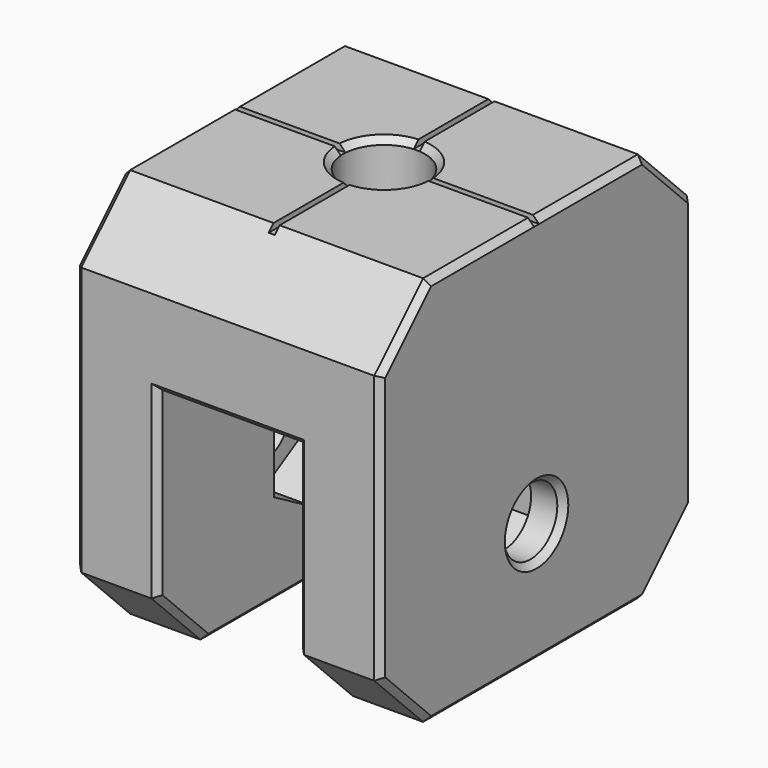
from build123d import *

# Parameters (mm, degrees)
F0_W      = 6.75
F0_H      = 32
F0_W_2    = 11.5
F0_R      = 3.35
F1_DEPTH  = 12
F2_DEPTH  = 20
F3_SIZE   = 5
F4_SIZE   = 5
F6_D      = 5.5
F8_DEPTH  = 4.1
F10_SIZE  = 0.5
F9_W      = 12.25
F9_H      = 0.5
F9_W_2    = 0.5
F9_H_2    = 15.75
F11_DEPTH = 0.5


# Not quite as in the source:
# - a pattern or mirror of a feature is missing from the dataset's text; its kind, count and spacing are read off the source's solid


with BuildPart() as f1:
    # F0 (on Top) → F1 (new body)
    with BuildSketch(Plane.XY):
        with Locations((9.125, 0)):
            Rectangle(F0_W, F0_H)
        Rectangle(F0_W_2, F0_H)
        Circle(F0_R, mode=Mode.SUBTRACT)
        with Locations((-9.125, 0)):
            Rectangle(F0_W, F0_H)
    extrude(amount=F1_DEPTH)

    # F0 (on Top) → F2 (join)
    with BuildSketch(Plane.XY):
        with Locations((9.125, 0)):
            Rectangle(F0_W, F0_H)
        with Locations((-9.125, 0)):
            Rectangle(F0_W, F0_H)
    extrude(amount=-F2_DEPTH)

    # F3
    f3_edges = [f1.edges().sort_by_distance(p)[0] for p in [
        (-9.125, -16, -20),
        (9.125, -16, -20),
        (9.125, 16, -20),
        (-9.125, 16, -20),
    ]]
    chamfer(f3_edges, length=F3_SIZE)

    # F4
    f4_edges = [f1.edges().sort_by_distance(p)[0] for p in [
        (0, -16, 12),
        (0, 16, 12),
    ]]
    chamfer(f4_edges, length=F4_SIZE)

    # F6 (through all)
    with Locations(Plane(origin=(-12.5, 0, 0), x_dir=(0, -1, 0), z_dir=(-1, 0, 0))):
        with Locations((0, -10)):
            Hole(F6_D / 2)

    # F7 (on face) → F8 (cut)
    with BuildSketch(Plane(origin=(5.75, 0, 0), x_dir=(0, -1, 0), z_dir=(-1, 0, 0))):
        Polygon((4.1, -12.3671361037), (4.1, -7.6328638963), (0, -5.2657277926), (-4.1, -7.6328638963), (-4.1, -12.3671361037), (0, -14.7342722074), align=None)
    f8 = extrude(amount=-F8_DEPTH, mode=Mode.SUBTRACT)

    # F8_copies: F8 across plane
    add(f8.mirror(Plane(origin=(0, 0, 0), x_dir=(0, 0, -1), z_dir=(-1, 0, 0))), mode=Mode.SUBTRACT)

    # F10
    f10_edges = [f1.edges().sort_by_distance(p)[0] for p in [
        (12.5, 0, 12),
        (12.5, -13.5, 9.5),
        (12.5, -16, -4),
        (12.5, -13.5, -17.5),
        (12.5, 0, -20),
        (12.5, 13.5, -17.5),
        (12.5, 16, -4),
        (12.5, 13.5, 9.5),
        (-12.5, -16, -4),
        (-12.5, -13.5, 9.5),
        (-12.5, -13.5, -17.5),
        (-12.5, 0, 12),
        (-12.5, 0, -20),
        (-12.5, 13.5, 9.5),
        (-12.5, 13.5, -17.5),
        (-12.5, 16, -4),
        (-12.5, 2.75, -10),
        (0, 16, 0),
        (0, -16, 0),
        (5.75, -16, -7.5),
        (5.75, -13.5, -17.5),
        (5.75, 0, -20),
        (5.75, 13.5, -17.5),
        (5.75, 16, -7.5),
        (-5.75, 16, -7.5),
        (-5.75, 13.5, -17.5),
        (-5.75, 0, -20),
        (-5.75, -13.5, -17.5),
        (-5.75, -16, -7.5),
        (-3.35, 0, 12),
        (-3.35, 0, 0),
        (12.5, 2.75, -10),
    ]]
    chamfer(f10_edges, length=F10_SIZE)

    # F9 (on face) → F11 (cut)
    with BuildSketch(Plane.XY.offset(12)):
        with Locations((-6.375, 0)):
            Rectangle(F9_W, F9_H)
        Rectangle(F9_W_2, F9_H)
        with Locations((0, -8.125)):
            Rectangle(F9_W_2, F9_H_2)
        with Locations((6.375, 0)):
            Rectangle(F9_W, F9_H)
        with Locations((0, 8.125)):
            Rectangle(F9_W_2, F9_H_2)
    extrude(amount=-F11_DEPTH, mode=Mode.SUBTRACT)


solid = f1.part
